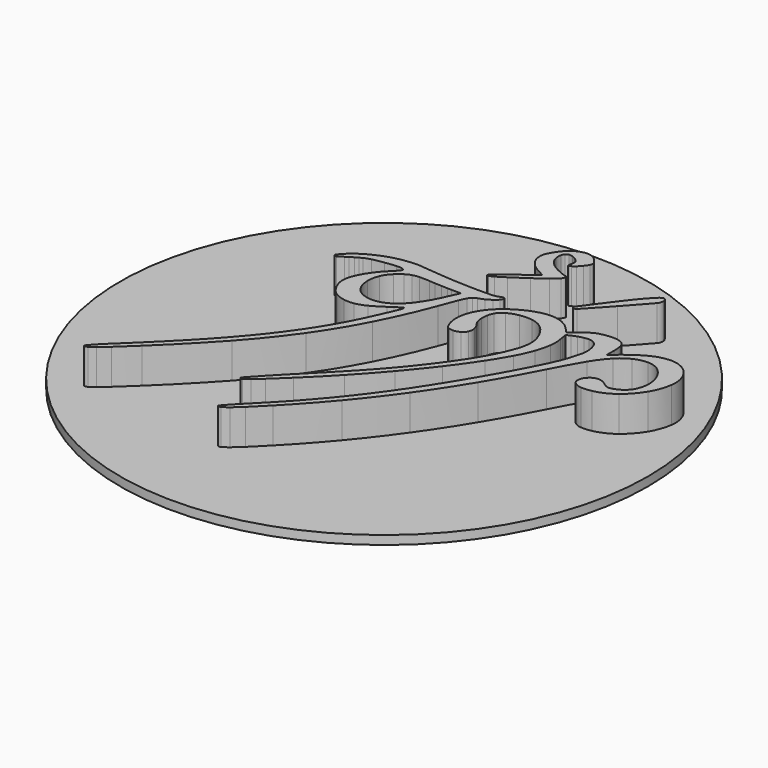
from build123d import *

# Parameters (mm, degrees)
F0_R     = 3810
F1_DEPTH = 635
F2_R     = 3810
F3_DEPTH = 508


# Not quite as in the source:
# - ends of sketch curves that miss each other by under 0.0002 mm in the source are joined


with BuildPart() as f1:
    # F0 (on Top) → F1 (new body)
    with BuildSketch(Plane.XY):
        with Locations((-347.4214971066, -304.5988678932)):
            Circle(F0_R)
    extrude(amount=F1_DEPTH)

    # F2 (on face) → F3 (cut)
    with BuildSketch(Plane.XY.offset(635)):
        with Locations((-347.4214971066, -304.5988678932)):
            Circle(F2_R)
        with BuildLine():
            ThreePointArc((-1581.3868549001, 1282.2209811115), (-1503.2529169774, 1306.0164401121), (-1423.5474955558, 1323.8540946765))
            ThreePointArc((-1423.5474955558, 1323.8540946765), (-1385.5996133276, 1330.3744256698), (-1347.5030944444, 1335.9611707107))
            ThreePointArc((-1347.5030944444, 1335.9611707107), (-1308.3932513381, 1340.7515216456), (-1269.1839223455, 1344.6445681803))
            ThreePointArc((-1269.1839223455, 1344.6445681803), (-1234.2604494419, 1347.3037085202), (-1199.2850033897, 1349.1579409968))
            ThreePointArc((-1199.2850033897, 1349.1579409968), (-1176.1406711826, 1349.2440700702), (-1153.0557085829, 1347.5851546569))
            ThreePointArc((-1153.0557085829, 1347.5851546569), (-942.7821024035, 1326.2716681229), (-732.1783163686, 1308.5149961677))
            ThreePointArc((-732.1783163686, 1308.5149961677), (-551.7847824466, 1297.2800673887), (-371.1541726444, 1290.9056203629))
            ThreePointArc((-371.1541726444, 1290.9056203629), (-227.6627695431, 1289.5935264588), (-84.184184977, 1291.9173474759))
            ThreePointArc((-84.184184977, 1291.9173474759), (-17.124748305, 1300.3369037518), (47.0942970332, 1321.4027822271))
            ThreePointArc((47.0942970332, 1321.4027822271), (57.2570501892, 1325.3353968084), (67.7248337943, 1328.3640142988))
            ThreePointArc((67.7248337943, 1328.3640142988), (74.5296240554, 1328.8720214868), (81.137583151, 1327.1696363557))
            ThreePointArc((81.137583151, 1327.1696363557), (85.9623933128, 1323.6757682427), (88.9301107329, 1318.5106428185))
            ThreePointArc((88.9301107329, 1318.5106428185), (90.8868072238, 1310.2536093179), (91.5442924, 1301.7934086))
            ThreePointArc((91.5442924, 1301.7934086), (87.178681512, 1279.6974371918), (74.7379009396, 1260.9219880721))
            ThreePointArc((74.7379009396, 1260.9219880721), (45.5929720834, 1233.7727582011), (14.3427902058, 1209.0759233015))
            ThreePointArc((14.3427902058, 1209.0759233015), (-23.8122473195, 1183.6666636769), (-63.9072810485, 1161.4444735658))
            ThreePointArc((-63.9072810485, 1161.4444735658), (-103.3121119937, 1144.0178204655), (-144.2328321828, 1130.5299171159))
            ThreePointArc((-144.2328321828, 1130.5299171159), (-171.7377754653, 1119.6023808604), (-196.2359559726, 1102.9959917443))
            ThreePointArc((-196.2359559726, 1102.9959917443), (-218.1850907956, 1080.5771871395), (-235.6880019255, 1054.5384574929))
            ThreePointArc((-235.6880019255, 1054.5384574929), (-259.532394517, 1007.2919366916), (-280.2155896126, 958.5785485054))
            ThreePointArc((-280.2155896126, 958.5785485054), (-328.2703011452, 833.0907609967), (-375.6024060102, 707.3286364392))
            ThreePointArc((-375.6024060102, 707.3286364392), (-533.4919588091, 319.476204387), (-713.9846991846, -58.3875156715))
            ThreePointArc((-713.9846991846, -58.3875156715), (-907.9905727664, -405.5737081844), (-1125.4299446204, -738.5851960837))
            ThreePointArc((-1125.4299446204, -738.5851960837), (-1382.348709027, -1080.6677495678), (-1660.1553584222, -1406.0155479962))
            ThreePointArc((-1660.1553584222, -1406.0155479962), (-2010.9931073266, -1777.7610135115), (-2375.3041004348, -2136.3127075228))
            ThreePointArc((-2375.3041004348, -2136.3127075228), (-2500.3712151609, -2254.3249767398), (-2626.0507673965, -2371.6848038552))
            ThreePointArc((-2626.0507673965, -2371.6848038552), (-2689.4906031459, -2428.5754251462), (-2754.8882888532, -2483.2041568489))
            ThreePointArc((-2754.8882888532, -2483.2041568489), (-2794.4275029918, -2513.0085213694), (-2835.815860898, -2540.1867009656))
            ThreePointArc((-2835.815860898, -2540.1867009656), (-2858.8615634172, -2548.1065842839), (-2883.0980908905, -2545.5729012714))
            ThreePointArc((-2883.0980908905, -2545.5729012714), (-2887.9447866422, -2540.539896041), (-2886.5671189952, -2533.6898066655))
            ThreePointArc((-2886.5671189952, -2533.6898066655), (-2862.4900609554, -2504.5766930043), (-2837.8339351947, -2475.952339881))
            ThreePointArc((-2837.8339351947, -2475.952339881), (-2805.2432394313, -2439.9773400951), (-2771.5884890426, -2404.9957475682))
            ThreePointArc((-2771.5884890426, -2404.9957475682), (-2729.6712298837, -2363.4174146923), (-2687.0619895237, -2322.5485143122))
            ThreePointArc((-2687.0619895237, -2322.5485143122), (-2373.6794331985, -2020.8251012943), (-2066.5701932223, -1712.7186923147))
            ThreePointArc((-2066.5701932223, -1712.7186923147), (-1824.7213003894, -1455.4040263283), (-1592.8581327055, -1189.056141334))
            ThreePointArc((-1592.8581327055, -1189.056141334), (-1404.2318361223, -953.0571029015), (-1226.6234587512, -708.6584732648))
            ThreePointArc((-1226.6234587512, -708.6584732648), (-1075.1051716918, -475.4285772029), (-937.5405092417, -233.7057211535))
            ThreePointArc((-937.5405092417, -233.7057211535), (-891.1478844517, -143.9973387574), (-846.6939622272, -53.312619264))
            ThreePointArc((-846.6939622272, -53.312619264), (-796.531156225, 53.7106430179), (-747.8133621504, 161.3993718448))
            ThreePointArc((-747.8133621504, 161.3993718448), (-701.5877265399, 266.2870781888), (-655.9939188483, 371.4509742006))
            ThreePointArc((-655.9939188483, 371.4509742006), (-647.8186309267, 397.4585702964), (-645.0557076, 424.5804564))
            ThreePointArc((-645.0557076, 424.5804564), (-647.4223607435, 428.835353551), (-652.2855556698, 429.0688743787))
            ThreePointArc((-652.2855556698, 429.0688743787), (-673.1634473495, 418.3713153544), (-693.7362743213, 407.0982091567))
            ThreePointArc((-693.7362743213, 407.0982091567), (-720.7400216104, 391.1988227444), (-747.1886466974, 374.392184386))
            ThreePointArc((-747.1886466974, 374.392184386), (-779.1831282315, 352.8665726577), (-810.7768147631, 330.7568963497))
            ThreePointArc((-810.7768147631, 330.7568963497), (-901.6108409821, 270.6549091833), (-996.4531708629, 217.101181503))
            ThreePointArc((-996.4531708629, 217.101181503), (-1074.1847374443, 183.805377338), (-1155.9797042042, 162.348668771))
            ThreePointArc((-1155.9797042042, 162.348668771), (-1228.4318923026, 155.7842152828), (-1300.8606689982, 162.6021174616))
            ThreePointArc((-1300.8606689982, 162.6021174616), (-1373.220407552, 182.6154659952), (-1441.2230515178, 214.4290850987))
            ThreePointArc((-1441.2230515178, 214.4290850987), (-1474.7992802983, 237.8535248845), (-1503.7732975246, 266.7771075403))
            ThreePointArc((-1503.7732975246, 266.7771075403), (-1533.3986047703, 305.9593416511), (-1558.8640839479, 347.9642928158))
            ThreePointArc((-1558.8640839479, 347.9642928158), (-1580.4234507662, 393.3611222597), (-1597.3018122301, 440.698203289))
            ThreePointArc((-1597.3018122301, 440.698203289), (-1606.8796102163, 483.8718764349), (-1610.007573562, 527.9844151957))
            ThreePointArc((-1610.007573562, 527.9844151957), (-1605.3693674163, 582.3918327556), (-1591.9026634637, 635.3099580104))
            ThreePointArc((-1591.9026634637, 635.3099580104), (-1566.7667780015, 699.6610346867), (-1536.4303523959, 761.7301497489))
            ThreePointArc((-1536.4303523959, 761.7301497489), (-1497.003870567, 828.4966452232), (-1452.6609926245, 892.1042037283))
            ThreePointArc((-1452.6609926245, 892.1042037283), (-1402.4781052033, 954.0067336684), (-1348.1202684426, 1012.2774044426))
            ThreePointArc((-1348.1202684426, 1012.2774044426), (-1306.7278760252, 1054.0943861612), (-1265.7644190671, 1096.3316364245))
            ThreePointArc((-1265.7644190671, 1096.3316364245), (-1251.2947004506, 1113.4391104933), (-1239.0868102707, 1132.2275592983))
            ThreePointArc((-1239.0868102707, 1132.2275592983), (-1236.7003295118, 1142.539281961), (-1240.2725112314, 1152.502538501))
            ThreePointArc((-1240.2725112314, 1152.502538501), (-1249.452202347, 1161.3942899507), (-1261.0847278151, 1166.6871478829))
            ThreePointArc((-1261.0847278151, 1166.6871478829), (-1304.293387135, 1174.1042932693), (-1348.1339811209, 1174.0363330119))
            ThreePointArc((-1348.1339811209, 1174.0363330119), (-1429.9277080269, 1165.6201835008), (-1511.4276602151, 1154.7204985614))
            ThreePointArc((-1511.4276602151, 1154.7204985614), (-1593.0913048497, 1141.166365117), (-1674.2691697065, 1124.9546513055))
            ThreePointArc((-1674.2691697065, 1124.9546513055), (-1722.7982155134, 1111.037665488), (-1769.0794901667, 1090.868523418))
            ThreePointArc((-1769.0794901667, 1090.868523418), (-1788.3945544077, 1080.6464113559), (-1807.5028127939, 1070.0427446063))
            ThreePointArc((-1807.5028127939, 1070.0427446063), (-1831.5497843425, 1056.2274665126), (-1855.4596850365, 1042.1762958866))
            ThreePointArc((-1855.4596850365, 1042.1762958866), (-1880.1238738478, 1027.3548110541), (-1904.6422360801, 1012.293319278))
            ThreePointArc((-1904.6422360801, 1012.293319278), (-1926.0796026322, 998.7674346203), (-1947.3220462824, 984.9374369156))
            ThreePointArc((-1947.3220462824, 984.9374369156), (-1987.6314619673, 959.4546547957), (-2028.9512708723, 935.6451070048))
            ThreePointArc((-2028.9512708723, 935.6451070048), (-2043.9563402996, 933.3458001328), (-2056.9108304246, 941.2590958175))
            ThreePointArc((-2056.9108304246, 941.2590958175), (-2061.9303527104, 955.8244775499), (-2056.664552669, 970.302639367))
            ThreePointArc((-2056.664552669, 970.302639367), (-2025.3824848007, 1006.7461575063), (-1992.6576651466, 1041.8998764067))
            ThreePointArc((-1992.6576651466, 1041.8998764067), (-1940.9473565929, 1089.9158399626), (-1884.4768739541, 1132.2310062487))
            ThreePointArc((-1884.4768739541, 1132.2310062487), (-1814.1296866827, 1176.1214074255), (-1741.0715241768, 1215.3336373532))
            ThreePointArc((-1741.0715241768, 1215.3336373532), (-1662.288316576, 1251.3058346182), (-1581.3868549001, 1282.2209811115))
        make_face(mode=Mode.SUBTRACT)
        with BuildLine():
            ThreePointArc((1401.4673238843, 1282.9707182861), (1421.0297078878, 1292.5324218972), (1441.2260464788, 1300.6700475562))
            ThreePointArc((1441.2260464788, 1300.6700475562), (1461.5536998367, 1307.3149783977), (1482.2570303976, 1312.6760132105))
            ThreePointArc((1482.2570303976, 1312.6760132105), (1508.9678427408, 1318.2811904791), (1535.8372114208, 1323.0689396881))
            ThreePointArc((1535.8372114208, 1323.0689396881), (1564.0763793713, 1327.2217503445), (1592.4278537334, 1330.5218018352))
            ThreePointArc((1592.4278537334, 1330.5218018352), (1617.8612073594, 1332.5543401434), (1643.3575970013, 1333.5139312002))
            ThreePointArc((1643.3575970013, 1333.5139312002), (1694.6516882424, 1331.0392818031), (1745.1964806694, 1321.9601053269))
            ThreePointArc((1745.1964806694, 1321.9601053269), (1780.6119775299, 1307.2686271925), (1810.0680725271, 1282.7240688507))
            ThreePointArc((1810.0680725271, 1282.7240688507), (1832.701186255, 1248.9081093545), (1845.4525915404, 1210.2664382479))
            ThreePointArc((1845.4525915404, 1210.2664382479), (1853.3029003793, 1152.466943025), (1855.5529633996, 1094.1801839327))
            Line((1855.5529633996, 1094.1801839327), (1854.2616458, 959.9534776))
            Line((1854.2616458, 959.9534776), (1969.8529564, 1057.0749496))
            ThreePointArc((1969.8529564, 1057.0749496), (2099.8550941354, 1154.7800309085), (2239.6785750326, 1237.8235920074))
            ThreePointArc((2239.6785750326, 1237.8235920074), (2360.1067423425, 1285.3191682549), (2487.832160063, 1306.4139584581))
            ThreePointArc((2487.832160063, 1306.4139584581), (2593.1866021258, 1297.2945867413), (2691.6091492974, 1258.6199936811))
            ThreePointArc((2691.6091492974, 1258.6199936811), (2775.8027769978, 1193.355397748), (2838.513377485, 1107.2425935833))
            ThreePointArc((2838.513377485, 1107.2425935833), (2881.978799797, 980.417060212), (2883.8040991912, 846.3624915114))
            ThreePointArc((2883.8040991912, 846.3624915114), (2845.8193681896, 693.4995560169), (2778.5379878127, 551.0806957083))
            ThreePointArc((2778.5379878127, 551.0806957083), (2679.502802854, 415.8391626373), (2557.433232634, 300.959833204))
            ThreePointArc((2557.433232634, 300.959833204), (2424.2153364302, 219.2397794821), (2276.0740116166, 169.4469747947))
            ThreePointArc((2276.0740116166, 169.4469747947), (2201.6811159997, 158.6093350923), (2126.507887897, 157.74730411))
            ThreePointArc((2126.507887897, 157.74730411), (2070.6556600392, 169.2702060614), (2020.611379221, 196.616475859))
            ThreePointArc((2020.611379221, 196.616475859), (1992.9515477762, 230.26655158), (1983.4762961549, 272.7825888158))
            ThreePointArc((1983.4762961549, 272.7825888158), (1992.0455237678, 322.3782632471), (2015.425844209, 366.9486911747))
            ThreePointArc((2015.425844209, 366.9486911747), (2039.901597252, 394.3158152117), (2068.9068348458, 416.8262176408))
            ThreePointArc((2068.9068348458, 416.8262176408), (2099.5457497783, 431.8975904479), (2132.7712996512, 439.7685637769))
            ThreePointArc((2132.7712996512, 439.7685637769), (2167.2615115265, 440.102112426), (2200.9836053782, 432.8559935564))
            ThreePointArc((2200.9836053782, 432.8559935564), (2235.4465911499, 417.9439807022), (2266.8468308537, 397.3505205876))
            ThreePointArc((2266.8468308537, 397.3505205876), (2293.7347297757, 377.9665819302), (2322.1503965284, 360.9006478335))
            ThreePointArc((2322.1503965284, 360.9006478335), (2344.1764325665, 351.8483715068), (2367.6391302905, 347.7750678836))
            ThreePointArc((2367.6391302905, 347.7750678836), (2392.9346498773, 348.6463247785), (2417.5841966012, 354.3928260048))
            ThreePointArc((2417.5841966012, 354.3928260048), (2453.7756186671, 367.8307197262), (2489.1216175752, 383.3567094377))
            ThreePointArc((2489.1216175752, 383.3567094377), (2581.2968894991, 451.3974371568), (2641.1090925374, 549.1129486191))
            ThreePointArc((2641.1090925374, 549.1129486191), (2668.3123099871, 673.7381551002), (2659.6221849761, 801.0014197435))
            ThreePointArc((2659.6221849761, 801.0014197435), (2615.8518432127, 919.8472908544), (2540.2990921868, 1021.4935699431))
            ThreePointArc((2540.2990921868, 1021.4935699431), (2446.2344473805, 1084.6571357324), (2335.1244382, 1106.8463004))
            ThreePointArc((2335.1244382, 1106.8463004), (2233.7565925294, 1095.509006043), (2137.398137692, 1062.0572114638))
            ThreePointArc((2137.398137692, 1062.0572114638), (2044.5377724734, 1006.5153241783), (1963.6242721747, 934.6755449808))
            ThreePointArc((1963.6242721747, 934.6755449808), (1866.1593388205, 818.0461913807), (1782.1102025121, 691.4066944516))
            ThreePointArc((1782.1102025121, 691.4066944516), (1661.1924763777, 478.5241977781), (1546.405756207, 262.2741973726))
            ThreePointArc((1546.405756207, 262.2741973726), (1348.6795268852, -107.8768361284), (1138.5477896414, -471.128955549))
            ThreePointArc((1138.5477896414, -471.128955549), (924.1565000256, -812.7857149809), (696.9096877956, -1146.0301489103))
            ThreePointArc((696.9096877956, -1146.0301489103), (462.3488980143, -1463.021640517), (215.6016995775, -1770.6223390439))
            ThreePointArc((215.6016995775, -1770.6223390439), (-42.0071272487, -2067.1312873222), (-311.118616322, -2353.2411803624))
            ThreePointArc((-311.118616322, -2353.2411803624), (-420.6032729075, -2464.1033389937), (-531.1062730869, -2573.9504835944))
            ThreePointArc((-531.1062730869, -2573.9504835944), (-595.0399229998, -2634.1147279533), (-661.6469104542, -2691.3052611536))
            ThreePointArc((-661.6469104542, -2691.3052611536), (-703.0170731352, -2722.623812464), (-746.6860065382, -2750.6481999436))
            ThreePointArc((-746.6860065382, -2750.6481999436), (-768.8970895677, -2755.2090468314), (-789.2538433094, -2745.2222453094))
            ThreePointArc((-789.2538433094, -2745.2222453094), (-791.4913681559, -2740.0234452241), (-789.5425716361, -2734.7096641304))
            ThreePointArc((-789.5425716361, -2734.7096641304), (-753.6410474532, -2694.8157274939), (-717.5569438909, -2655.0868577575))
            ThreePointArc((-717.5569438909, -2655.0868577575), (-674.8045786826, -2608.9396473213), (-631.357849888, -2563.4455651154))
            ThreePointArc((-631.357849888, -2563.4455651154), (-579.1229946463, -2510.0605890343), (-526.4046163845, -2457.1530435879))
            ThreePointArc((-526.4046163845, -2457.1530435879), (-288.9597585813, -2212.503636074), (-60.3235442394, -1959.6027171447))
            ThreePointArc((-60.3235442394, -1959.6027171447), (153.3142201604, -1705.0529517958), (357.0680456646, -1442.5247515909))
            ThreePointArc((357.0680456646, -1442.5247515909), (560.3926309984, -1159.425853853), (753.3653387112, -869.1718154138))
            ThreePointArc((753.3653387112, -869.1718154138), (959.170559981, -537.812078169), (1156.3596214556, -201.2537046362))
            ThreePointArc((1156.3596214556, -201.2537046362), (1319.107182044, 95.7336019966), (1472.3988964967, 397.7102221025))
            ThreePointArc((1472.3988964967, 397.7102221025), (1555.5441103728, 596.2119079365), (1615.4519454267, 802.9172451101))
            ThreePointArc((1615.4519454267, 802.9172451101), (1624.9144013601, 919.992196362), (1600.6967019921, 1034.9251608327))
            ThreePointArc((1600.6967019921, 1034.9251608327), (1546.3026335494, 1105.5089174286), (1461.2973822, 1132.2463004))
            ThreePointArc((1461.2973822, 1132.2463004), (1428.6376626356, 1130.6217882847), (1396.3003565647, 1125.7643241609))
            ThreePointArc((1396.3003565647, 1125.7643241609), (1357.3638799666, 1116.8006304592), (1318.978461656, 1105.7120466049))
            ThreePointArc((1318.978461656, 1105.7120466049), (1281.7805955783, 1092.7127406905), (1245.353735494, 1077.6878583604))
            ThreePointArc((1245.353735494, 1077.6878583604), (1217.9416306527, 1063.5799131355), (1192.2984513461, 1046.4660329953))
            ThreePointArc((1192.2984513461, 1046.4660329953), (1191.2031905397, 1045.0581388843), (1190.9683729675, 1043.2899111159))
            ThreePointArc((1190.9683729675, 1043.2899111159), (1193.0431888809, 1027.9402452812), (1195.1740102418, 1012.5982538118))
            ThreePointArc((1195.1740102418, 1012.5982538118), (1197.7904773384, 994.8326812187), (1200.6340041061, 977.1020347863))
            ThreePointArc((1200.6340041061, 977.1020347863), (1204.1893068127, 956.3127865763), (1207.9093319822, 935.552381124))
            ThreePointArc((1207.9093319822, 935.552381124), (1217.30121464, 842.1595289851), (1211.4980994415, 748.475183722))
            ThreePointArc((1211.4980994415, 748.475183722), (1190.3201064789, 640.1292895761), (1158.4053993347, 534.4467867542))
            ThreePointArc((1158.4053993347, 534.4467867542), (1107.5724041694, 408.190820148), (1046.9680455939, 286.3233741293))
            ThreePointArc((1046.9680455939, 286.3233741293), (962.0759010626, 138.4260097847), (871.269444434, -5.9155776398))
            ThreePointArc((871.269444434, -5.9155776398), (731.20996688, -210.8214128686), (583.9440708529, -410.6108383584))
            ThreePointArc((583.9440708529, -410.6108383584), (414.0891341412, -626.7202825227), (238.6212380281, -838.2977122908))
            ThreePointArc((238.6212380281, -838.2977122908), (48.7653071851, -1055.6005386451), (-146.5029615795, -1268.0531122144))
            ThreePointArc((-146.5029615795, -1268.0531122144), (-347.6786457288, -1476.2109946872), (-553.9840550154, -1679.2859515254))
            ThreePointArc((-553.9840550154, -1679.2859515254), (-667.8952820396, -1787.9992450228), (-782.452618779, -1896.0314828619))
            ThreePointArc((-782.452618779, -1896.0314828619), (-843.7410987398, -1951.501252085), (-906.934089171, -2004.7912053193))
            ThreePointArc((-906.934089171, -2004.7912053193), (-945.3546571853, -2034.3036226892), (-985.3704115874, -2061.6141007669))
            ThreePointArc((-985.3704115874, -2061.6141007669), (-1002.9891609215, -2065.7721431208), (-1019.3183945342, -2057.9576939341))
            ThreePointArc((-1019.3183945342, -2057.9576939341), (-1022.2089368601, -2051.1913763201), (-1019.6196998746, -2044.3041440441))
            ThreePointArc((-1019.6196998746, -2044.3041440441), (-954.5041528064, -1973.3447814228), (-889.2173640612, -1902.5429394474))
            ThreePointArc((-889.2173640612, -1902.5429394474), (-813.4431271465, -1821.4638208763), (-736.7837132962, -1741.2211095365))
            ThreePointArc((-736.7837132962, -1741.2211095365), (-644.9221987946, -1646.7405531807), (-552.4404268231, -1552.8670465987))
            ThreePointArc((-552.4404268231, -1552.8670465987), (-370.6521098895, -1368.156870422), (-190.272082071, -1182.0711725873))
            ThreePointArc((-190.272082071, -1182.0711725873), (-59.798112287, -1043.8707715883), (68.0593718723, -903.2461957387))
            ThreePointArc((68.0593718723, -903.2461957387), (175.0036303768, -780.5186826794), (279.0439208579, -655.3199012057))
            ThreePointArc((279.0439208579, -655.3199012057), (384.1624040133, -522.959660907), (486.4881485654, -388.4287326159))
            ThreePointArc((486.4881485654, -388.4287326159), (600.6342186029, -229.4597116893), (709.2897767516, -66.6885694858))
            ThreePointArc((709.2897767516, -66.6885694858), (794.4612169537, 74.4016800469), (871.4771598884, 220.1040376461))
            ThreePointArc((871.4771598884, 220.1040376461), (926.426737207, 341.9609360313), (972.9211233079, 467.2878366353))
            ThreePointArc((972.9211233079, 467.2878366353), (996.9764783792, 564.7090359963), (1005.4085456108, 664.7012868515))
            ThreePointArc((1005.4085456108, 664.7012868515), (1001.8540986655, 717.0888649174), (990.7264076843, 768.404234091))
            ThreePointArc((990.7264076843, 768.404234091), (970.9825913929, 825.0079125818), (945.7768063103, 879.3996680644))
            ThreePointArc((945.7768063103, 879.3996680644), (915.4050288881, 930.9572898421), (880.1118958497, 979.2794157997))
            ThreePointArc((880.1118958497, 979.2794157997), (844.385770447, 1017.3259035147), (803.4461902686, 1049.6962919344))
            ThreePointArc((803.4461902686, 1049.6962919344), (735.3321002326, 1085.1518642384), (660.9211569116, 1104.1160014659))
            ThreePointArc((660.9211569116, 1104.1160014659), (572.529712803, 1109.3092579397), (484.365527304, 1101.1181762276))
            ThreePointArc((484.365527304, 1101.1181762276), (402.1769868612, 1080.3851634823), (324.2611309971, 1047.0095266361))
            ThreePointArc((324.2611309971, 1047.0095266361), (269.9133589971, 1006.8805362446), (230.1254023184, 952.2825986498))
            ThreePointArc((230.1254023184, 952.2825986498), (213.1514117465, 912.7297880311), (202.0183303951, 871.1534032754))
            ThreePointArc((202.0183303951, 871.1534032754), (195.9390923049, 825.2950587189), (195.2051992194, 779.0413426682))
            ThreePointArc((195.2051992194, 779.0413426682), (199.7319088371, 734.8579135839), (209.5150152403, 691.5340474034))
            ThreePointArc((209.5150152403, 691.5340474034), (223.5092811003, 656.2423979337), (243.9443057497, 624.2463108423))
            ThreePointArc((243.9443057497, 624.2463108423), (271.9846927982, 578.9238941505), (289.4833900343, 528.5832505925))
            ThreePointArc((289.4833900343, 528.5832505925), (292.6629803681, 481.5680217026), (281.1419182436, 435.8755012187))
            ThreePointArc((281.1419182436, 435.8755012187), (256.5762051234, 397.6164803769), (220.8518771676, 369.4917775688))
            ThreePointArc((220.8518771676, 369.4917775688), (174.1813560398, 351.1051037827), (124.4115368, 344.8463004))
            ThreePointArc((124.4115368, 344.8463004), (100.3548369591, 345.7404266046), (76.4308862444, 348.4178976327))
            ThreePointArc((76.4308862444, 348.4178976327), (60.9444587836, 352.649893545), (46.8792247592, 360.3899492397))
            ThreePointArc((46.8792247592, 360.3899492397), (34.4332746027, 371.5375114024), (24.6981195571, 385.1167799372))
            ThreePointArc((24.6981195571, 385.1167799372), (12.3236172681, 408.6820043544), (1.3482219866, 432.9304842289))
            ThreePointArc((1.3482219866, 432.9304842289), (-27.2759060052, 535.6491468807), (-29.8085916992, 642.2514449839))
            ThreePointArc((-29.8085916992, 642.2514449839), (-7.0388637808, 755.184580307), (37.4372241922, 861.4589006334))
            ThreePointArc((37.4372241922, 861.4589006334), (108.0396220996, 969.0294410811), (195.966608857, 1062.970726449))
            ThreePointArc((195.966608857, 1062.970726449), (305.8262096453, 1149.2034508039), (426.2506902731, 1219.9364608607))
            ThreePointArc((426.2506902731, 1219.9364608607), (522.9098183892, 1262.3865724025), (623.3277150358, 1294.9633277209))
            ThreePointArc((623.3277150358, 1294.9633277209), (711.6258865028, 1311.2858394443), (801.4000739946, 1313.1798287957))
            ThreePointArc((801.4000739946, 1313.1798287957), (880.5427275355, 1300.880098084), (955.9694089615, 1273.9420493859))
            ThreePointArc((955.9694089615, 1273.9420493859), (1024.6920327525, 1233.4041028387), (1084.4694143577, 1180.5572583653))
            Line((1084.4694143577, 1180.5572583653), (1157.0333476, 1102.8772964))
            Line((1157.0333476, 1102.8772964), (1256.4206012, 1186.317922))
            ThreePointArc((1256.4206012, 1186.317922), (1278.2236602969, 1203.8766886759), (1300.7251403932, 1220.5310291576))
            ThreePointArc((1300.7251403932, 1220.5310291576), (1325.9501116582, 1237.8288110282), (1351.7044424232, 1254.3281101872))
            ThreePointArc((1351.7044424232, 1254.3281101872), (1376.3578957766, 1269.0455128933), (1401.4673238843, 1282.9707182861))
        make_face(mode=Mode.SUBTRACT)
        with BuildLine():
            ThreePointArc((-84.6405095171, 2657.4488760829), (-48.5327730135, 2689.2308814984), (-7.4169840542, 2714.1979878964))
            ThreePointArc((-7.4169840542, 2714.1979878964), (35.3638135563, 2732.7873091448), (79.7234428284, 2747.2089121855))
            ThreePointArc((79.7234428284, 2747.2089121855), (117.8158051312, 2754.2917897463), (156.5544739354, 2755.006516162))
            ThreePointArc((156.5544739354, 2755.006516162), (191.0985713192, 2749.4410456238), (223.9581247768, 2737.4194429696))
            ThreePointArc((223.9581247768, 2737.4194429696), (255.3600041952, 2718.9778486301), (283.1988478542, 2695.5008558542))
            ThreePointArc((283.1988478542, 2695.5008558542), (295.4767396193, 2682.5632432234), (307.0612520889, 2669.0012544407))
            ThreePointArc((307.0612520889, 2669.0012544407), (317.5490846683, 2655.2628259142), (327.2302919281, 2640.9445426666))
            ThreePointArc((327.2302919281, 2640.9445426666), (334.7414267599, 2628.2969011801), (341.483547748, 2615.2231179845))
            ThreePointArc((341.483547748, 2615.2231179845), (344.5163640559, 2606.5021352719), (345.5442924, 2597.3262506))
            ThreePointArc((345.5442924, 2597.3262506), (342.5931859525, 2575.6254546975), (333.9541949255, 2555.5008079651))
            ThreePointArc((333.9541949255, 2555.5008079651), (313.9463373561, 2524.419432868), (292.0328845382, 2494.6508776513))
            ThreePointArc((292.0328845382, 2494.6508776513), (267.0411553246, 2464.9235381827), (240.1321489122, 2436.9198505537))
            ThreePointArc((240.1321489122, 2436.9198505537), (217.1549808416, 2417.4898184613), (191.6854110544, 2401.4655427779))
            ThreePointArc((191.6854110544, 2401.4655427779), (178.0654510839, 2394.6687901704), (164.0800672487, 2388.6597788782))
            ThreePointArc((164.0800672487, 2388.6597788782), (158.3082216131, 2388.4081888037), (153.619262204, 2391.7832685514))
            ThreePointArc((153.619262204, 2391.7832685514), (150.6602050657, 2398.3781886186), (150.3789451914, 2405.6010565395))
            ThreePointArc((150.3789451914, 2405.6010565395), (153.9884719756, 2427.4498716236), (158.0874772468, 2449.2121682306))
            ThreePointArc((158.0874772468, 2449.2121682306), (161.1197819849, 2468.4892034482), (162.5484686452, 2487.9509041922))
            ThreePointArc((162.5484686452, 2487.9509041922), (161.5696020081, 2502.3275136786), (157.7571475324, 2516.2239267323))
            ThreePointArc((157.7571475324, 2516.2239267323), (151.3312503029, 2528.8636712272), (142.4627522655, 2539.9273503453))
            ThreePointArc((142.4627522655, 2539.9273503453), (128.6929852499, 2552.6796341766), (113.8248399759, 2564.1323844246))
            ThreePointArc((113.8248399759, 2564.1323844246), (82.4381523258, 2583.448015659), (48.9851985008, 2598.9114471088))
            ThreePointArc((48.9851985008, 2598.9114471088), (21.8228342202, 2605.5995506515), (-6.1433957383, 2604.9556189718))
            ThreePointArc((-6.1433957383, 2604.9556189718), (-28.1444856461, 2597.3212554064), (-46.0829294944, 2582.4705432357))
            ThreePointArc((-46.0829294944, 2582.4705432357), (-60.2921980032, 2560.4668487514), (-68.5093718943, 2535.5963022064))
            ThreePointArc((-68.5093718943, 2535.5963022064), (-72.4401886016, 2493.1889394315), (-67.9069984795, 2450.8417334526))
            ThreePointArc((-67.9069984795, 2450.8417334526), (-55.0604652752, 2409.0832184193), (-34.7693362035, 2370.3911360978))
            ThreePointArc((-34.7693362035, 2370.3911360978), (-5.072269669, 2331.7428515387), (30.3960017318, 2298.3122176161))
            ThreePointArc((30.3960017318, 2298.3122176161), (75.7470458016, 2265.7623712004), (124.3098605687, 2238.2330647372))
            ThreePointArc((124.3098605687, 2238.2330647372), (150.2817928194, 2225.6096640223), (176.4982693028, 2213.502315847))
            ThreePointArc((176.4982693028, 2213.502315847), (201.1817564437, 2202.7577961507), (226.1200193102, 2192.6186503325))
            ThreePointArc((226.1200193102, 2192.6186503325), (247.1338062349, 2184.6291695309), (268.3127517992, 2177.0883936029))
            ThreePointArc((268.3127517992, 2177.0883936029), (278.4603797189, 2174.5127613909), (288.8938596, 2173.6463004))
            ThreePointArc((288.8938596, 2173.6463004), (305.5529062211, 2166.0079002514), (310.6362714962, 2148.4002772251))
            ThreePointArc((310.6362714962, 2148.4002772251), (302.2693463689, 2121.5581943016), (286.1906303442, 2098.4935508524))
            ThreePointArc((286.1906303442, 2098.4935508524), (238.2183160283, 2052.1857747453), (186.6181670487, 2009.9580855283))
            ThreePointArc((186.6181670487, 2009.9580855283), (101.5904495771, 1947.470221548), (15.1951678076, 1886.8872109413))
            ThreePointArc((15.1951678076, 1886.8872109413), (-93.8771744856, 1812.7029366762), (-203.4175140831, 1739.2114649157))
            ThreePointArc((-203.4175140831, 1739.2114649157), (-264.0364941049, 1700.2826702336), (-325.9363339747, 1663.4245428917))
            ThreePointArc((-325.9363339747, 1663.4245428917), (-361.5783839953, 1644.4177785974), (-398.3047648176, 1627.6015425965))
            ThreePointArc((-398.3047648176, 1627.6015425965), (-410.6114798403, 1628.7537652999), (-416.4557076, 1639.6454126))
            ThreePointArc((-416.4557076, 1639.6454126), (-414.5987250006, 1648.2729001589), (-409.3566814798, 1655.3724005412))
            ThreePointArc((-409.3566814798, 1655.3724005412), (-377.1814736317, 1683.4798921219), (-344.7404260741, 1711.2801352041))
            ThreePointArc((-344.7404260741, 1711.2801352041), (-305.6331791397, 1743.8088189259), (-265.8873705658, 1775.5540977558))
            ThreePointArc((-265.8873705658, 1775.5540977558), (-219.332757468, 1811.5046581839), (-172.3186123742, 1846.8521471585))
            Line((-172.3186123742, 1846.8521471585), (71.8185254, 2027.9552024))
            Line((71.8185254, 2027.9552024), (-40.9442412, 2089.9664322))
            ThreePointArc((-40.9442412, 2089.9664322), (-84.3538260687, 2116.6301327402), (-125.0056508558, 2147.3347609367))
            ThreePointArc((-125.0056508558, 2147.3347609367), (-158.3616409569, 2179.0359448983), (-187.3235334486, 2214.7962006966))
            ThreePointArc((-187.3235334486, 2214.7962006966), (-209.141174612, 2250.9115181431), (-225.5299844944, 2289.7925226675))
            ThreePointArc((-225.5299844944, 2289.7925226675), (-235.3522778446, 2329.0803713374), (-238.6557075999, 2369.4424798))
            ThreePointArc((-238.6557075999, 2369.4424798), (-234.0061789414, 2413.490876822), (-220.2625271803, 2455.5977816386))
            ThreePointArc((-220.2625271803, 2455.5977816386), (-193.226976581, 2509.7294423309), (-161.6895214458, 2561.3680580503))
            ThreePointArc((-161.6895214458, 2561.3680580503), (-125.2103395793, 2611.0486505236), (-84.6405095171, 2657.4488760829))
        make_face(mode=Mode.SUBTRACT)
        with BuildLine():
            ThreePointArc((1227.929619306, 2176.0367237859), (1298.168208688, 2262.3409844735), (1371.6620478569, 2345.8906131705))
            ThreePointArc((1371.6620478569, 2345.8906131705), (1405.6308789436, 2381.4534452547), (1441.1215984824, 2415.4976127561))
            ThreePointArc((1441.1215984824, 2415.4976127561), (1462.4687642417, 2430.7351151125), (1486.880392147, 2440.3244449297))
            ThreePointArc((1486.880392147, 2440.3244449297), (1503.3656981228, 2439.5605113872), (1516.5839740625, 2429.6799162528))
            ThreePointArc((1516.5839740625, 2429.6799162528), (1527.7744031677, 2409.6689701796), (1533.8336342162, 2387.5567690256))
            ThreePointArc((1533.8336342162, 2387.5567690256), (1530.6449041219, 2342.424675565), (1508.791302683, 2302.8078317168))
            ThreePointArc((1508.791302683, 2302.8078317168), (1357.4672874915, 2132.1216557136), (1204.621391992, 1962.7969367321))
            ThreePointArc((1204.621391992, 1962.7969367321), (1048.5149279303, 1792.6364559744), (891.1941306522, 1623.5980459014))
            ThreePointArc((891.1941306522, 1623.5980459014), (864.3809881168, 1611.7226098539), (837.1982318507, 1622.7257184507))
            ThreePointArc((837.1982318507, 1622.7257184507), (831.0593687985, 1636.0635872629), (835.0710453449, 1650.1877115458))
            ThreePointArc((835.0710453449, 1650.1877115458), (935.3396072685, 1787.0729466706), (1035.9962458196, 1923.6730682721))
            ThreePointArc((1035.9962458196, 1923.6730682721), (1131.0954222505, 2050.5146747966), (1227.929619306, 2176.0367237859))
        make_face(mode=Mode.SUBTRACT)
        with BuildLine():
            Line((-367.981484, 1106.8463004), (-500.1685958, 1106.998548))
            ThreePointArc((-500.1685958, 1106.998548), (-532.5795666369, 1107.276036733), (-564.9828678504, 1108.033729856))
            ThreePointArc((-564.9828678504, 1108.033729856), (-609.1041883215, 1109.5254258792), (-653.2157365854, 1111.2825216756))
            ThreePointArc((-653.2157365854, 1111.2825216756), (-700.6538479939, 1113.4564690865), (-748.0781840896, 1115.9126473129))
            ThreePointArc((-748.0781840896, 1115.9126473129), (-791.8272682444, 1118.4750790869), (-835.5557076461, 1121.3685211409))
            ThreePointArc((-835.5557076461, 1121.3685211409), (-907.0476362215, 1124.704902623), (-978.6173719723, 1124.7185433133))
            ThreePointArc((-978.6173719723, 1124.7185433133), (-1028.0552630617, 1120.268096101), (-1076.4608931292, 1109.276887685))
            ThreePointArc((-1076.4608931292, 1109.276887685), (-1119.4246892942, 1092.8051869752), (-1159.3957305061, 1070.0121931553))
            ThreePointArc((-1159.3957305061, 1070.0121931553), (-1206.8376571711, 1035.3201515737), (-1251.5792397059, 997.2089335984))
            ThreePointArc((-1251.5792397059, 997.2089335984), (-1307.0002481437, 933.7728726256), (-1347.2248497979, 859.7620389281))
            ThreePointArc((-1347.2248497979, 859.7620389281), (-1372.1019608205, 776.0351595764), (-1380.0393446884, 689.0520634665))
            ThreePointArc((-1380.0393446884, 689.0520634665), (-1370.6537412629, 606.2730053293), (-1344.2195804619, 527.2685955641))
            ThreePointArc((-1344.2195804619, 527.2685955641), (-1303.6185465949, 463.728983282), (-1246.9673952748, 413.9658142949))
            ThreePointArc((-1246.9673952748, 413.9658142949), (-1152.0388111485, 370.5683040377), (-1048.4921118623, 357.4206236984))
            ThreePointArc((-1048.4921118623, 357.4206236984), (-939.8539124339, 374.3788305061), (-839.2176723995, 418.6754069944))
            ThreePointArc((-839.2176723995, 418.6754069944), (-730.3710200575, 499.7820309807), (-638.9702029959, 600.1402310919))
            ThreePointArc((-638.9702029959, 600.1402310919), (-546.8353548336, 737.8606837527), (-469.8651503696, 884.5963000193))
            Line((-469.8651503696, 884.5963000193), (-367.981484, 1106.8463004))
        make_face()
    extrude(amount=-F3_DEPTH, mode=Mode.SUBTRACT)


solid = f1.part
